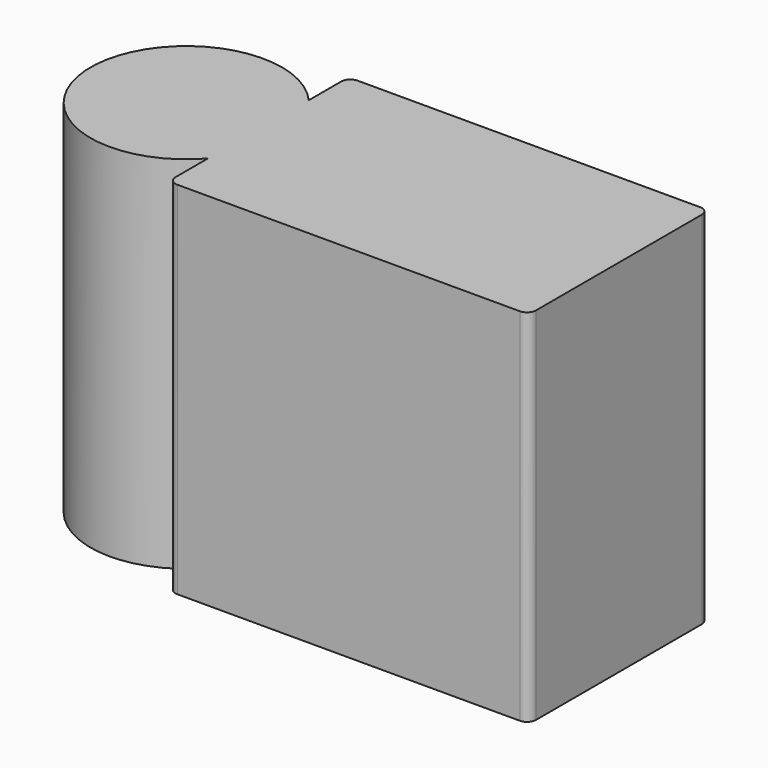
from build123d import *

# Parameters (mm, degrees)
F1_DEPTH = 101.6


with BuildPart() as f1:
    # F0 (on Top) → F1 (new body)
    with BuildSketch(Plane.XY):
        with BuildLine():
            ThreePointArc((50.8, 29.21), (50.0560512242, 31.0060512242), (48.26, 31.75))
            Line((48.26, 31.75), (-48.26, 31.75))
            ThreePointArc((-48.26, 31.75), (-50.0560512242, 31.0060512242), (-50.8, 29.21))
            Line((-50.8, 29.21), (-50.8, 17.7601451641))
            ThreePointArc((-50.8, 17.7601451641), (-45.8543003634, 9.4852294714), (-44.1325, 0))
            ThreePointArc((-44.1325, 0), (-45.8543003634, -9.4852294714), (-50.8, -17.7601451641))
            Line((-50.8, -17.7601451641), (-50.8, -29.21))
            ThreePointArc((-50.8, -29.21), (-50.0560512242, -31.0060512242), (-48.26, -31.75))
            Line((-48.26, -31.75), (48.26, -31.75))
            ThreePointArc((48.26, -31.75), (50.0560512242, -31.0060512242), (50.8, -29.21))
            Line((50.8, -29.21), (50.8, 29.21))
        make_face()
        with BuildLine():
            ThreePointArc((-44.1325, 0), (-45.8543003634, 9.4852294714), (-50.8, 17.7601451641))
            Line((-50.8, 17.7601451641), (-50.8, -17.7601451641))
            ThreePointArc((-50.8, -17.7601451641), (-45.8543003634, -9.4852294714), (-44.1325, 0))
        make_face()
        with BuildLine():
            Line((-50.8, -17.7601451641), (-50.8, 17.7601451641))
            ThreePointArc((-50.8, 17.7601451641), (-98.1075, 0), (-50.8, -17.7601451641))
        make_face()
    extrude(amount=-F1_DEPTH)


solid = f1.part
